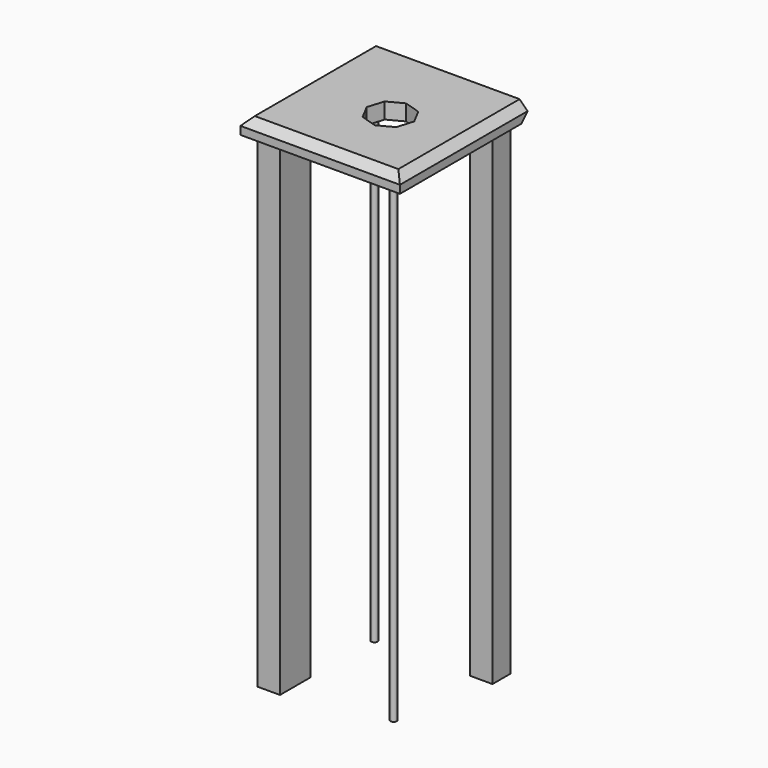
from build123d import *

# Parameters (mm, degrees)
F0_W     = 100
F0_H     = 100
F1_DEPTH = 10
F3_DEPTH = 28
F4_R     = 2
F5_DEPTH = 305
F6_R     = 2
F7_DEPTH = 305
F8_W     = 14
F8_H     = 24
F8_H_2   = 14
F9_DEPTH = 305
F10_SIZE = 4.99999


# Not quite as in the source:
# - a fillet or chamfer is up to 0.001 mm smaller than in the source, because OpenCascade refuses the exact size


with BuildPart() as f1:
    # F0 (on Top) → F1 (new body)
    with BuildSketch(Plane.XY):
        with Locations((-5.6718036532, 2.052295208)):
            Rectangle(F0_W, F0_H)
    extrude(amount=F1_DEPTH)

    # F2 (on Top) → F3 (cut)
    with BuildSketch(Plane.XY):
        Polygon((-8.8692104674, -10.7118982853), (1.3029770516, -13.8459347822), (10.7118982853, -8.8692104674), (13.8459347822, 1.3029770516), (8.8692104674, 10.7118982853), (-1.3029770516, 13.8459347822), (-10.7118982853, 8.8692104674), (-13.8459347822, -1.3029770516), align=None)
    extrude(amount=F3_DEPTH, mode=Mode.SUBTRACT)

    # F4 (on Top) → F5 (join)
    with BuildSketch(Plane.XY):
        with Locations((24.3281963468, -27.947704792)):
            Circle(F4_R)
    extrude(amount=-F5_DEPTH)

    # F6 (on Top) → F7 (join)
    with BuildSketch(Plane.XY):
        with Locations((-35.6718036532, 32.052295208)):
            Circle(F6_R)
    extrude(amount=-F7_DEPTH)

    # F8 (on Top) → F9 (join)
    with BuildSketch(Plane.XY):
        with Locations((-42.6718036532, -29.947704792)):
            Rectangle(F8_W, F8_H)
        with Locations((31.3281963468, 39.052295208)):
            Rectangle(F8_W, F8_H_2)
    extrude(amount=-F9_DEPTH)

    # F10 (size 5 in the source; OpenCascade refuses exactly that, so slightly less here)
    f10_edges = [f1.edges().sort_by_distance(p)[0] for p in [
        (-55.671804, 2.052295, 10),
        (-5.671804, -47.947705, 10),
        (-5.671804, 52.052295, 0),
        (44.328196, 2.052295, 10),
    ]]
    chamfer(f10_edges, length=F10_SIZE)


solid = f1.part
